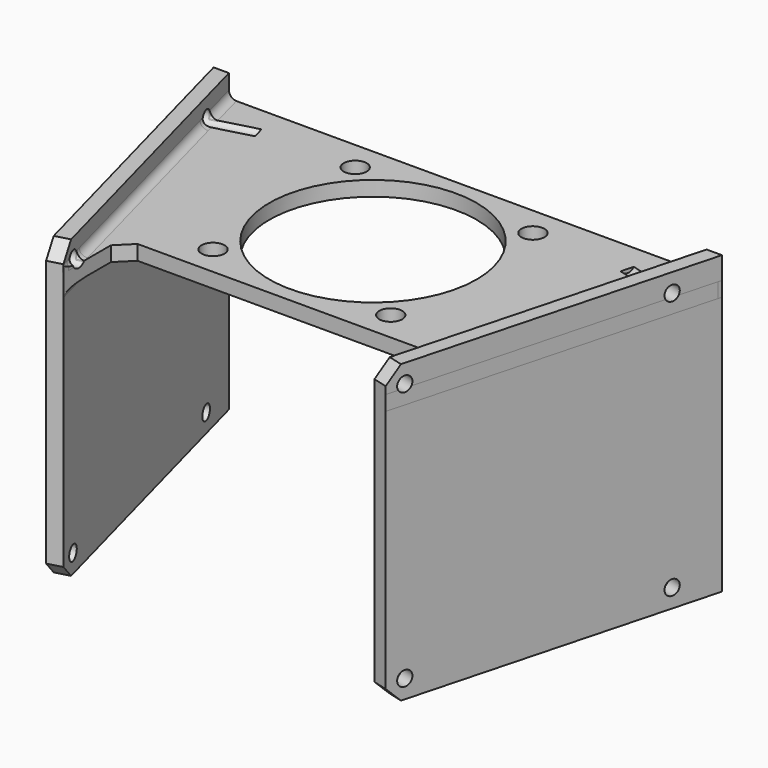
from build123d import *

# Parameters (mm, degrees)
F0_W          = 32
F0_H          = 32
F0_R          = 1.55
F0_R_2        = 14
F1_DEPTH      = 2
F3_DEPTH      = 35
F3_DEPTH_BACK = 5
F4_R          = 1
F5_DEPTH      = 8
F6_SIZE       = 2
F7_T4_DEPTH   = 38.2727780192
F7_S6_R       = 1
F7_T7_DEPTH   = 21
F7_S8_R       = 1
F7_T9_DEPTH   = 21
F7_T13_DEPTH  = 10.1204030002
F7_S15_R      = 1
F7_T16_DEPTH  = 7
F7_T20_DEPTH  = 4.1363890096
F7_S23_R      = 1
F7_T24_DEPTH  = 4
F7_T28_DEPTH  = 45.9840139906
F7_T34_DEPTH  = 45.9840139906
F7_T40_DEPTH  = 10.1204030002
F7_S42_R      = 1
F7_T43_DEPTH  = 7
F7_T47_DEPTH  = 4.1363890096
F7_S49_R      = 1
F7_T50_DEPTH  = 4
F7_T55_DEPTH  = 38.2727780192
F7_S56_R      = 1
F7_T57_DEPTH  = 21
F7_S58_R      = 1
F7_T59_DEPTH  = 21


# Not quite as in the source:
# - a fillet or chamfer that OpenCascade refuses, or shapes differently, is made with other operations: its cross-section is extruded or revolved along the edge and cut away or added
# - a pattern or mirror of a feature is missing from the dataset's text; its kind, count and spacing are read off the source's solid


with BuildPart() as f1:
    # F0 (on Top) → F1 (new body)
    with BuildSketch(Plane.XY):
        Rectangle(F0_W, F0_H)
        with Locations((-12, -12)):
            Circle(F0_R, mode=Mode.SUBTRACT)
        with Locations((12, -12)):
            Circle(F0_R, mode=Mode.SUBTRACT)
        Circle(F0_R_2, mode=Mode.SUBTRACT)
        with Locations((-12, 12)):
            Circle(F0_R, mode=Mode.SUBTRACT)
        with Locations((12, 12)):
            Circle(F0_R, mode=Mode.SUBTRACT)
        Polygon((-16, -16), (-16, 16), (-32.2534734714, 16), (-34.3244184429, 16), (-34.1856914348, 15.4822637571), (-22.9318516526, -26.5176380902), (-21, -26), (-21, -16), align=None)
        Polygon((32.2534734714, 16), (16, 16), (16, -16), (21, -16), (21, -26), (22.9318516526, -26.5176380902), (34.1856914348, 15.4822637571), (34.3244184429, 16), align=None)
    extrude(amount=F1_DEPTH)

    # F2 (on face) → F3 (join, two sides)
    with BuildSketch(Plane(origin=(0, 0, 0), x_dir=(1, 0, 0), z_dir=(0, 0, -1))) as f3_sk:
        Polygon((-21, 26), (-22.9318516526, 26.5176380902), (-34.3244184429, -16), (-32.2538660821, -16), align=None)
        Polygon((22.9318516526, 26.5176380902), (21, 26), (32.2538660821, -16), (34.3244184429, -16), align=None)
    extrude(amount=F3_DEPTH)
    extrude(f3_sk.sketch, amount=-F3_DEPTH_BACK)

    # F4 (on face) → F5 (cut)
    with BuildSketch(Plane(origin=(28.0251183923, -7.509307841, 0), x_dir=(0.2588190451, 0.9659258263, 0), z_dir=(0.9659258263, -0.2588190451, 0))):
        with Locations((-17.1788715364, 2.5)):
            Circle(F4_R)
        with Locations((-17.1788715364, -32.5)):
            Circle(F4_R)
        with Locations((17.8211284636, 2.5)):
            Circle(F4_R)
        with Locations((17.8211284636, -32.5)):
            Circle(F4_R)
    f5 = extrude(amount=-F5_DEPTH, mode=Mode.SUBTRACT)

    # F5_copies: F5 across plane
    add(f5.mirror(Plane(origin=(0, 0, 0), x_dir=(0, 0, -1), z_dir=(-1, 0, 0))), mode=Mode.SUBTRACT)

    # F6
    f6_edges = [f1.edges().sort_by_distance(p)[0] for p in [
        (21.965926, -26.258819, -35),
        (21.965926, -26.258819, 5),
        (-21.965926, -26.258819, 5),
        (-21.965926, -26.258819, -35),
        (-21, -16, 1),
        (21, -16, 1),
    ]]
    chamfer(f6_edges, length=F6_SIZE)

    # F7: fillet of radius 1 on 8 edges, made by hand


with BuildPart() as f7_tool2:
    # F7_s3 → F7_t4 (new body)
    with BuildSketch(Plane(origin=(-4.8697477679, -18.1741460897, 0), x_dir=(0, 0, 1), z_dir=(0.2588190451, 0.9659258263, 0))):
        with BuildLine():
            ThreePointArc((3.0009656854, 27.0141375247), (2.2928932188, 26.7208443059), (1.9996, 26.0127718393))
            Line((1.9996, 26.0127718393), (1.8994634315, 26.0127718393))
            ThreePointArc((1.8994634315, 26.0127718393), (1.8998634315, 26.513254682), (1.8998634315, 27.0137375247))
            Line((1.8998634315, 27.0137375247), (2, 27.1138740933))
            ThreePointArc((2, 27.1138740933), (2.5004828427, 27.1138740933), (3.0009656854, 27.1142740933))
            Line((3.0009656854, 27.1142740933), (3.0009656854, 27.0141375247))
        make_face()
    extrude(amount=F7_T4_DEPTH)

    split(bisect_by=Plane.YZ.offset(21), keep=Keep.TOP)

    # F7_s6 → F7_t7 (cut, symmetric)
    with BuildSketch(Plane(origin=(25.6936269793, -6.8845865997, 0), x_dir=(0, 0, 1), z_dir=(0.9659258263, -0.2588190451, 0))):
        with Locations((2.5, 17.1788715364)):
            Circle(F7_S6_R)
    extrude(amount=F7_T7_DEPTH, both=True, mode=Mode.SUBTRACT)

    # F7_s8 → F7_t9 (cut, symmetric)
    with BuildSketch(Plane(origin=(25.6936269793, -6.8845865997, 0), x_dir=(0, 0, 1), z_dir=(0.9659258263, -0.2588190451, 0))):
        with Locations((2.5, -17.8211284636)):
            Circle(F7_S8_R)
    extrude(amount=F7_T9_DEPTH, both=True, mode=Mode.SUBTRACT)


with BuildPart() as f1_1:
    add(f1.part)

    # F7_t1: union F7_tool2
    add(f7_tool2.part)


with BuildPart() as f7_tool11:
    # F7_s12 → F7_t13 (new body)
    with BuildSketch(Plane(origin=(4.1889188107, 15.6332578304, 0), x_dir=(0, 0, 1), z_dir=(0.2588190451, 0.9659258263, 0))):
        with BuildLine():
            ThreePointArc((3.0009656854, 27.0141375247), (2.2928932188, 26.7208443059), (1.9996, 26.0127718393))
            Line((1.9996, 26.0127718393), (1.8994634315, 26.0127718393))
            ThreePointArc((1.8994634315, 26.0127718393), (1.8998634315, 26.513254682), (1.8998634315, 27.0137375247))
            Line((1.8998634315, 27.0137375247), (2, 27.1138740933))
            ThreePointArc((2, 27.1138740933), (2.5004828427, 27.1138740933), (3.0009656854, 27.1142740933))
            Line((3.0009656854, 27.1142740933), (3.0009656854, 27.0141375247))
        make_face()
    extrude(amount=F7_T13_DEPTH)

    split(bisect_by=Plane.XZ.offset(-16), keep=Keep.TOP)

    # F7_s15 → F7_t16 (cut, symmetric)
    with BuildSketch(Plane(origin=(25.6936269793, -6.8845865997, 0), x_dir=(0, 0, 1), z_dir=(0.9659258263, -0.2588190451, 0))):
        with Locations((2.5, -17.8211284636)):
            Circle(F7_S15_R)
    extrude(amount=F7_T16_DEPTH, both=True, mode=Mode.SUBTRACT)


with BuildPart() as f1_2:
    add(f1_1.part)

    # F7_t10: union F7_tool11
    add(f7_tool11.part)


with BuildPart() as f7_tool18:
    # F7_s19 → F7_t20 (new body)
    with BuildSketch(Plane(origin=(-5.0932667397, -19.0083302492, 0), x_dir=(0, 0, 1), z_dir=(0.2588190451, 0.9659258263, 0))):
        with BuildLine():
            ThreePointArc((3.0009656854, 27.0141375247), (2.2928932188, 26.7208443059), (1.9996, 26.0127718393))
            Line((1.9996, 26.0127718393), (1.8994634315, 26.0127718393))
            ThreePointArc((1.8994634315, 26.0127718393), (1.8998634315, 26.513254682), (1.8998634315, 27.0137375247))
            Line((1.8998634315, 27.0137375247), (2, 27.1138740933))
            ThreePointArc((2, 27.1138740933), (2.5004828427, 27.1138740933), (3.0009656854, 27.1142740933))
            Line((3.0009656854, 27.1142740933), (3.0009656854, 27.0141375247))
        make_face()
    extrude(amount=F7_T20_DEPTH)

    split(bisect_by=Plane.YZ.offset(21), keep=Keep.TOP)

    split(bisect_by=Plane(origin=(-2.9348619375, -10.953053864, 11.3394357682), x_dir=(-0.9659258263, 0.2588190451, 0), z_dir=(0.1830127019, 0.6830127019, -0.7071067812)), keep=Keep.TOP)

    # F7_s23 → F7_t24 (cut, symmetric)
    with BuildSketch(Plane(origin=(25.6936269793, -6.8845865997, 0), x_dir=(0, 0, 1), z_dir=(0.9659258263, -0.2588190451, 0))):
        with Locations((2.5, 17.1788715364)):
            Circle(F7_S23_R)
    extrude(amount=F7_T24_DEPTH, both=True, mode=Mode.SUBTRACT)


with BuildPart() as f1_3:
    add(f1_2.part)

    # F7_t17: union F7_tool18
    add(f7_tool18.part)


with BuildPart() as f7_tool26:
    # F7_s27 → F7_t28 (new body)
    with BuildSketch(Plane(origin=(-6.8082718513, 25.4088164608, 0), x_dir=(0, 0, 1), z_dir=(0.2588190451, -0.9659258263, 0))):
        with BuildLine():
            ThreePointArc((-1.0009656854, 27.0141375247), (-0.2928932188, 26.7208443059), (0.0004, 26.0127718393))
            Line((0.0004, 26.0127718393), (0.1005365685, 26.0127718393))
            ThreePointArc((0.1005365685, 26.0127718393), (0.1001365685, 26.513254682), (0.1001365685, 27.0137375247))
            Line((0.1001365685, 27.0137375247), (0, 27.1138740933))
            ThreePointArc((0, 27.1138740933), (-0.5004828427, 27.1138740933), (-1.0009656854, 27.1142740933))
            Line((-1.0009656854, 27.1142740933), (-1.0009656854, 27.0141375247))
        make_face()
    extrude(amount=F7_T28_DEPTH)

    split(bisect_by=Plane.XZ.offset(-16), keep=Keep.TOP)

    split(bisect_by=Plane.YZ.offset(-21), keep=Keep.BOTTOM)


with BuildPart() as f1_4:
    add(f1_3.part)

    # F7_t25: union F7_tool26
    add(f7_tool26.part)


with BuildPart() as f7_tool32:
    # F7_s33 → F7_t34 (new body)
    with BuildSketch(Plane(origin=(-5.0932667397, -19.0083302492, 0), x_dir=(0, 0, 1), z_dir=(0.2588190451, 0.9659258263, 0))):
        with BuildLine():
            ThreePointArc((0.0004, 26.0127718393), (-0.2928932188, 26.7208443059), (-1.0009656854, 27.0141375247))
            Line((-1.0009656854, 27.0141375247), (-1.0009656854, 27.1142740933))
            ThreePointArc((-1.0009656854, 27.1142740933), (-0.5004828427, 27.1138740933), (0, 27.1138740933))
            Line((0, 27.1138740933), (0.1001365685, 27.0137375247))
            ThreePointArc((0.1001365685, 27.0137375247), (0.1001365685, 26.513254682), (0.1005365685, 26.0127718393))
            Line((0.1005365685, 26.0127718393), (0.0004, 26.0127718393))
        make_face()
    extrude(amount=F7_T34_DEPTH)

    split(bisect_by=Plane.XZ.offset(-16), keep=Keep.TOP)

    split(bisect_by=Plane.YZ.offset(21), keep=Keep.TOP)


with BuildPart() as f1_5:
    add(f1_4.part)

    # F7_t31: union F7_tool32
    add(f7_tool32.part)


with BuildPart() as f7_tool38:
    # F7_s39 → F7_t40 (new body)
    with BuildSketch(Plane(origin=(-6.8082718513, 25.4088164608, 0), x_dir=(0, 0, 1), z_dir=(0.2588190451, -0.9659258263, 0))):
        with BuildLine():
            ThreePointArc((3.0009656854, 27.0141375247), (2.2928932188, 26.7208443059), (1.9996, 26.0127718393))
            Line((1.9996, 26.0127718393), (1.8994634315, 26.0127718393))
            ThreePointArc((1.8994634315, 26.0127718393), (1.8998634315, 26.513254682), (1.8998634315, 27.0137375247))
            Line((1.8998634315, 27.0137375247), (2, 27.1138740933))
            ThreePointArc((2, 27.1138740933), (2.5004828427, 27.1138740933), (3.0009656854, 27.1142740933))
            Line((3.0009656854, 27.1142740933), (3.0009656854, 27.0141375247))
        make_face()
    extrude(amount=F7_T40_DEPTH)

    split(bisect_by=Plane.XZ.offset(-16), keep=Keep.TOP)

    # F7_s42 → F7_t43 (cut, symmetric)
    with BuildSketch(Plane(origin=(-25.6936269793, -6.8845865997, 0), x_dir=(0, 0, 1), z_dir=(-0.9659258263, -0.2588190451, 0))):
        with Locations((2.5, 17.8211284636)):
            Circle(F7_S42_R)
    extrude(amount=F7_T43_DEPTH, both=True, mode=Mode.SUBTRACT)


with BuildPart() as f1_6:
    add(f1_5.part)

    # F7_t37: union F7_tool38
    add(f7_tool38.part)


with BuildPart() as f7_tool45:
    # F7_s46 → F7_t47 (new body)
    with BuildSketch(Plane(origin=(4.0226904861, -15.0128852773, 0), x_dir=(0, 0, 1), z_dir=(0.2588190451, -0.9659258263, 0))):
        with BuildLine():
            ThreePointArc((3.0009656854, 27.0141375247), (2.2928932188, 26.7208443059), (1.9996, 26.0127718393))
            Line((1.9996, 26.0127718393), (1.8994634315, 26.0127718393))
            ThreePointArc((1.8994634315, 26.0127718393), (1.8998634315, 26.513254682), (1.8998634315, 27.0137375247))
            Line((1.8998634315, 27.0137375247), (2, 27.1138740933))
            ThreePointArc((2, 27.1138740933), (2.5004828427, 27.1138740933), (3.0009656854, 27.1142740933))
            Line((3.0009656854, 27.1142740933), (3.0009656854, 27.0141375247))
        make_face()
    extrude(amount=F7_T47_DEPTH)

    split(bisect_by=Plane(origin=(2.9348619375, -10.953053864, 11.3394357682), x_dir=(-0.9659258263, -0.2588190451, 0), z_dir=(-0.1830127019, 0.6830127019, -0.7071067812)), keep=Keep.TOP)

    # F7_s49 → F7_t50 (cut, symmetric)
    with BuildSketch(Plane(origin=(-25.6936269793, -6.8845865997, 0), x_dir=(0, 0, 1), z_dir=(-0.9659258263, -0.2588190451, 0))):
        with Locations((2.5, -17.1788715364)):
            Circle(F7_S49_R)
    extrude(amount=F7_T50_DEPTH, both=True, mode=Mode.SUBTRACT)

    split(bisect_by=Plane.YZ.offset(-21), keep=Keep.BOTTOM)


with BuildPart() as f1_7:
    add(f1_6.part)

    # F7_t44: union F7_tool45
    add(f7_tool45.part)


with BuildPart() as f7_tool53:
    # F7_s54 → F7_t55 (new body)
    with BuildSketch(Plane(origin=(-5.0359760925, 18.7945186429, 0), x_dir=(0, 0, 1), z_dir=(0.2588190451, -0.9659258263, 0))):
        with BuildLine():
            ThreePointArc((3.0009656854, 27.0141375247), (2.2928932188, 26.7208443059), (1.9996, 26.0127718393))
            Line((1.9996, 26.0127718393), (1.8994634315, 26.0127718393))
            ThreePointArc((1.8994634315, 26.0127718393), (1.8998634315, 26.513254682), (1.8998634315, 27.0137375247))
            Line((1.8998634315, 27.0137375247), (2, 27.1138740933))
            ThreePointArc((2, 27.1138740933), (2.5004828427, 27.1138740933), (3.0009656854, 27.1142740933))
            Line((3.0009656854, 27.1142740933), (3.0009656854, 27.0141375247))
        make_face()
    extrude(amount=F7_T55_DEPTH)

    # F7_s56 → F7_t57 (cut, symmetric)
    with BuildSketch(Plane(origin=(-25.6936269793, -6.8845865997, 0), x_dir=(0, 0, 1), z_dir=(-0.9659258263, -0.2588190451, 0))):
        with Locations((2.5, 17.8211284636)):
            Circle(F7_S56_R)
    extrude(amount=F7_T57_DEPTH, both=True, mode=Mode.SUBTRACT)

    # F7_s58 → F7_t59 (cut, symmetric)
    with BuildSketch(Plane(origin=(-25.6936269793, -6.8845865997, 0), x_dir=(0, 0, 1), z_dir=(-0.9659258263, -0.2588190451, 0))):
        with Locations((2.5, -17.1788715364)):
            Circle(F7_S58_R)
    extrude(amount=F7_T59_DEPTH, both=True, mode=Mode.SUBTRACT)

    split(bisect_by=Plane.YZ.offset(-21), keep=Keep.BOTTOM)


with BuildPart() as f1_8:
    add(f1_7.part)

    # F7_t52: union F7_tool53
    add(f7_tool53.part)


solid = f1_8.part
